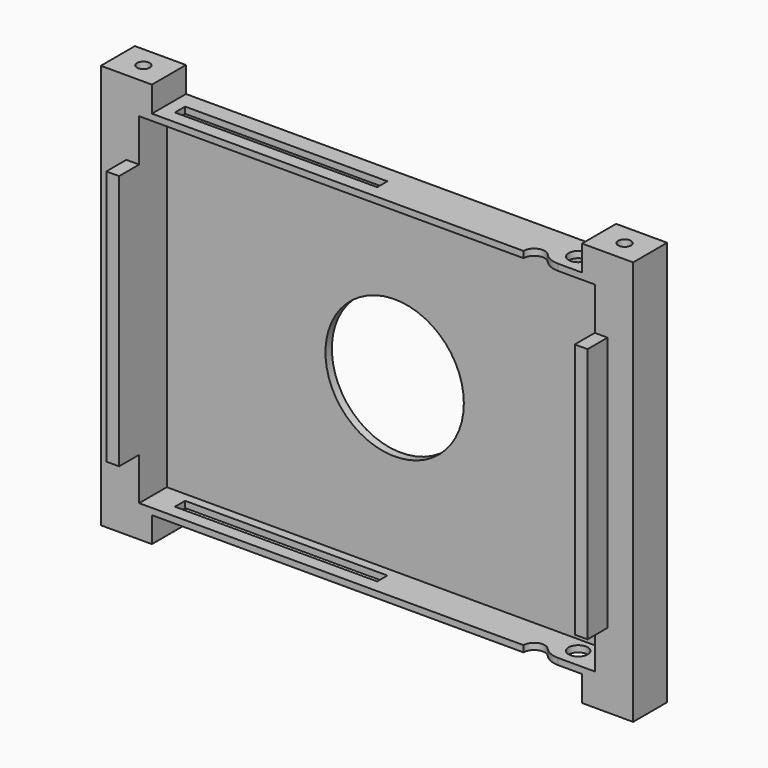
from build123d import *

# Parameters (mm, degrees)
F0_R      = 16.25
F1_DEPTH  = 15.875
F2_W      = 139.2096877098
F2_H      = 115.5483946204
F2_W_2    = 113
F2_H_2    = 80
F3_DEPTH  = 5.875
F4_W      = 107
F4_H      = 80
F5_DEPTH  = 14
F6_W      = 120.5911301091
F6_H      = 13.1527084535
F6_W_2    = 121.3300417974
F6_H_2    = 15.8128053223
F7_DEPTH  = 5.875
F8_R      = 1.5
F8_W      = 89
F8_H      = 3
F9_DEPTH  = 100
F10_W     = 42.4407012761
F10_H     = 10
F11_DEPTH = 1.5
F12_W     = 42.5221920013
F12_H     = 10
F13_DEPTH = 1.5
F14_R     = 2.5
F15_DEPTH = 95.5
F16_R     = 2.25
F17_DEPTH = 200
F18_R     = 5
F19_R     = 1.5
F20_DEPTH = 106.2
F21_R     = 1.5
F22_DEPTH = 121.8


with BuildPart() as f1:
    # F0 (on Front) → F1 (new body)
    with BuildSketch(Plane.XZ):
        Polygon((-50.5, 47.5), (-62.5, 47.5), (-62.5, -47.5), (-50.5, -47.5), (-50.5, -41.5), (50.5, -41.5), (50.5, -47.5), (62.5, -47.5), (62.5, 47.5), (50.5, 47.5), (50.5, 41.5), (-50.5, 41.5), align=None)
        Circle(F0_R, mode=Mode.SUBTRACT)
    extrude(amount=F1_DEPTH)

    # F2 (on face) → F3 (cut)
    with BuildSketch(Plane.XZ.offset(15.875)):
        Rectangle(F2_W, F2_H)
        Rectangle(F2_W_2, F2_H_2, mode=Mode.SUBTRACT)
    extrude(amount=-F3_DEPTH, mode=Mode.SUBTRACT)

    # F4 (on face) → F5 (cut)
    with BuildSketch(Plane.XZ.offset(15.875)):
        Rectangle(F4_W, F4_H)
    extrude(amount=-F5_DEPTH, mode=Mode.SUBTRACT)

    # F6 (on face) → F7 (cut)
    with BuildSketch(Plane.XZ.offset(15.875)):
        with Locations((0.0607829645, 36.5763542267)):
            Rectangle(F6_W, F6_H)
        with Locations((1.0213727103, -37.9064026611)):
            Rectangle(F6_W_2, F6_H_2)
    extrude(amount=-F7_DEPTH, mode=Mode.SUBTRACT)

    # F8 (on face) → F9 (cut)
    with BuildSketch(Plane.XY.offset(41.5)):
        with Locations((46, -5.5)):
            Circle(F8_R)
        with Locations((-3, -5.5)):
            Rectangle(F8_W, F8_H)
    extrude(amount=-F9_DEPTH, mode=Mode.SUBTRACT)

    # F10 (on face) → F11 (join)
    with BuildSketch(Plane.XY.offset(41.5)):
        with Locations((21.220350638, -5)):
            Rectangle(F10_W, F10_H)
    extrude(amount=-F11_DEPTH)

    # F12 (on face) → F13 (join)
    with BuildSketch(Plane(origin=(0, 0, -41.5), x_dir=(1, 0, 0), z_dir=(0, 0, -1))):
        with Locations((21.2610960007, 5)):
            Rectangle(F12_W, F12_H)
    extrude(amount=-F13_DEPTH)

    # F14 (on face) → F15 (cut)
    with BuildSketch(Plane(origin=(0, 0, -41.5), x_dir=(1, 0, 0), z_dir=(0, 0, -1))):
        with Locations((39.25, 10)):
            Circle(F14_R)
    extrude(amount=-F15_DEPTH, mode=Mode.SUBTRACT)

    # F16 (on face) → F17 (cut)
    with BuildSketch(Plane.XY.offset(41.5)):
        with Locations((46, -5.5)):
            Circle(F16_R)
    extrude(amount=-F17_DEPTH, mode=Mode.SUBTRACT)

    # F18
    f18_edges = [f1.edges().sort_by_distance(p)[0] for p in [
        (41.75, -10, -40.75),
        (41.75, -10, 40.75),
    ]]
    fillet(f18_edges, radius=F18_R)

    # F19 (on face) → F20 (cut)
    with BuildSketch(Plane.XY.offset(47.5)):
        with Locations((-56.5, -5)):
            Circle(F19_R)
    extrude(amount=-F20_DEPTH, mode=Mode.SUBTRACT)

    # F21 (on face) → F22 (cut)
    with BuildSketch(Plane.XY.offset(47.5)):
        with Locations((56.5, -5)):
            Circle(F21_R)
    extrude(amount=-F22_DEPTH, mode=Mode.SUBTRACT)


solid = f1.part
